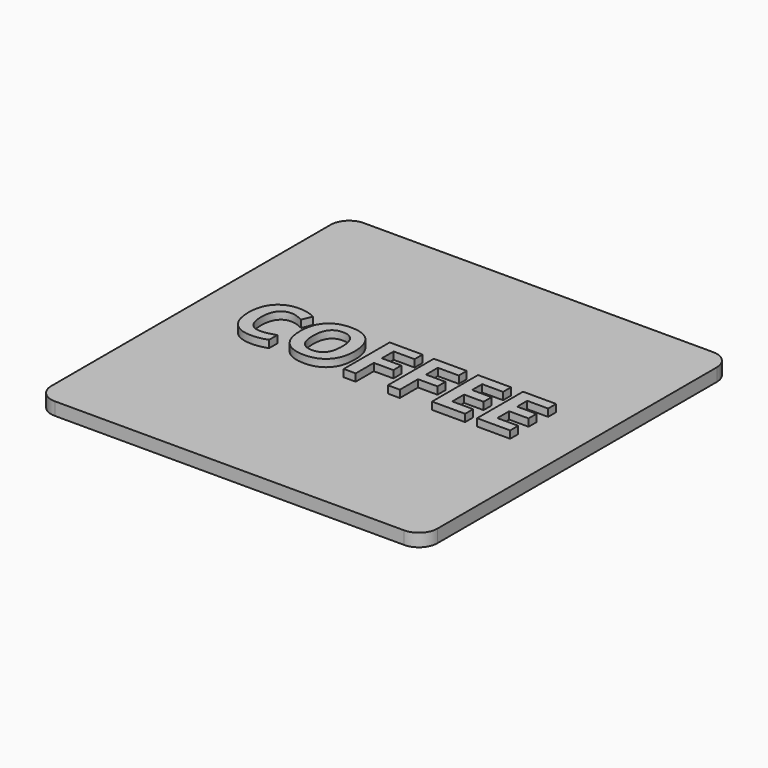
from build123d import *

# Parameters (mm, degrees)
F1_DEPTH     = 3.5
F2_TEXT_SIZE = 21.8775370679
F3_DEPTH     = 2


# Not quite as in the source:
# - Text() gives the source's letters only with a copy of the font that has no kerning and outlines rounded to 1/6400 em; it was checked with that copy


with BuildPart() as f1:
    # F0 (on Top) → F1 (new body)
    with BuildSketch(Plane.XY):
        with BuildLine():
            Line((-47.5, -52.5), (47.5, -52.5))
            ThreePointArc((47.5, -52.5), (51.0355339059, -51.0355339059), (52.5, -47.5))
            Line((52.5, -47.5), (52.5, 47.5))
            ThreePointArc((52.5, 47.5), (51.0355339059, 51.0355339059), (47.5, 52.5))
            Line((47.5, 52.5), (-47.5, 52.5))
            ThreePointArc((-47.5, 52.5), (-51.0355339059, 51.0355339059), (-52.5, 47.5))
            Line((-52.5, 47.5), (-52.5, -47.5))
            ThreePointArc((-52.5, -47.5), (-51.0355339059, -51.0355339059), (-47.5, -52.5))
        make_face()
    extrude(amount=F1_DEPTH)

    # F2 (on face) → F3 (join)
    with BuildSketch(Plane.XY.offset(3.5)):
        with Locations((-39.8262285929, -5.561829306)):
            Text('COFFEE', F2_TEXT_SIZE, font='Open Sans', font_style=FontStyle.BOLD, text_align=(TextAlign.LEFT, TextAlign.BOTTOM))
    extrude(amount=F3_DEPTH)


solid = f1.part
